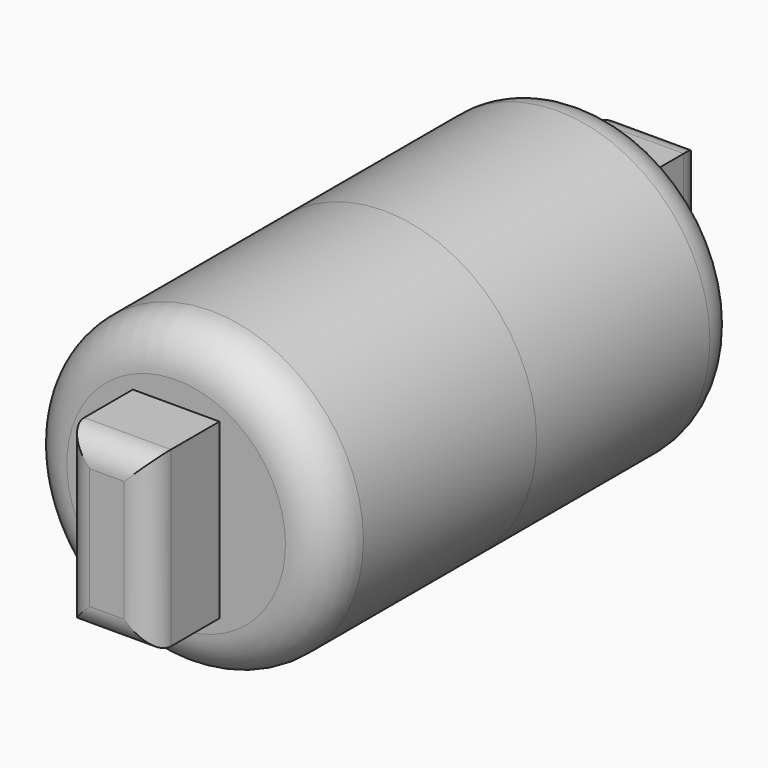
from build123d import *

# Parameters (mm, degrees)
F0_R        = 44.7584797017
F1_DEPTH    = 76.2
F2_DEPTH    = 25.4
F4_R        = 12.7
F3_W        = 25.4
F3_H        = 50.8
F5_DEPTH    = 25.4
F6_R        = 7.62
F7_T        = 2.54
F7_T3_DEPTH = 30.48
F7_T5_DEPTH = 55.88


# Not quite as in the source:
# - a shell that OpenCascade refuses in one call is made with other operations: the cavity is built on its own and cut out


with BuildPart() as f1:
    # F0 (on Front) → F1 (new body)
    with BuildSketch(Plane.XZ):
        Circle(F0_R)
    extrude(amount=F1_DEPTH)

    # F0 (on Front) → F2 (join)
    with BuildSketch(Plane.XZ):
        Circle(F0_R)
    extrude(amount=F2_DEPTH)

    # F4
    f4_edges = [f1.edges().sort_by_distance(p)[0] for p in [
        (-44.75848, 0, 0),
    ]]
    fillet(f4_edges, radius=F4_R)

    # F3 (on face) → F5 (join)
    with BuildSketch(Plane(origin=(0, 0, 0), x_dir=(-1, 0, 0), z_dir=(0, 1, 0))):
        Rectangle(F3_W, F3_H)
    extrude(amount=F5_DEPTH)

    # F6
    f6_edges = [f1.edges().sort_by_distance(p)[0] for p in [
        (-12.7, 25.4, 0),
        (0, 25.4, 25.4),
        (12.7, 25.4, 0),
        (0, 25.4, -25.4),
    ]]
    fillet(f6_edges, radius=F6_R)

    # F7: shell of thickness 2.54, made by hand


with BuildPart() as f7_core1:
    # F7_t2: copy of F1
    add(f1.part)

    # the walls: a layer under each face that stays
    f7_faces = [f7_core1.faces().sort_by_distance(p)[0] for p in [
        (0, 8.89, -25.4),
        (12.7, 8.89, 0),
        (0, 23.1681536726, -23.1681536726),
        (-21.3723198011, 0, -21.3723198011),
        (-12.7, 8.89, 0),
        (0, 8.89, 25.4),
        (10.4681536726, 23.1681536726, 0),
        (0, 25.4, 0),
        (-10.4681536726, 23.1681536726, 0),
        (-41.0387358228, -3.7197438789, 0),
        (0, 23.1681536726, 23.1681536726),
        (-44.7584797017, -44.45, 0),
    ]]
    thicken(f7_faces, amount=-F7_T, mode=Mode.SUBTRACT)

    # F7_s4 → F7_t3 (cut)
    with BuildSketch(Plane.YZ.offset(-15.24)):
        Polygon((0.0254, -25.4254), (0, -22.86), (-2.54, -22.86), (-2.54, -25.4), align=None)
        Polygon((0.0254, 25.4254), (-2.54, 25.4), (-2.54, 22.86), (0, 22.86), align=None)
    extrude(amount=F7_T3_DEPTH, mode=Mode.SUBTRACT)

    # F7_s6 → F7_t5 (cut)
    with BuildSketch(Plane.XY.offset(-27.94)):
        Polygon((12.7254, 0.0254), (10.16, 0), (10.16, -2.54), (12.7, -2.54), align=None)
        Polygon((-12.7254, 0.0254), (-12.7, -2.54), (-10.16, -2.54), (-10.16, 0), align=None)
    extrude(amount=F7_T5_DEPTH, mode=Mode.SUBTRACT)


with BuildPart() as f1_1:
    add(f1.part)

    # what is left inside the walls is the cavity
    f7_cavity = [f7_core1.part.solids().sort_by_distance(p)[0] for p in [
        (-42.19308, -55.033333, 0),
    ]]
    add(f7_cavity, mode=Mode.SUBTRACT)

    # F8: F1 across face


with BuildPart() as f1_2:
    add(f1_1.part)
    add(f1_1.part.mirror(Plane.XZ.offset(76.2)))


solid = f1_2.part
